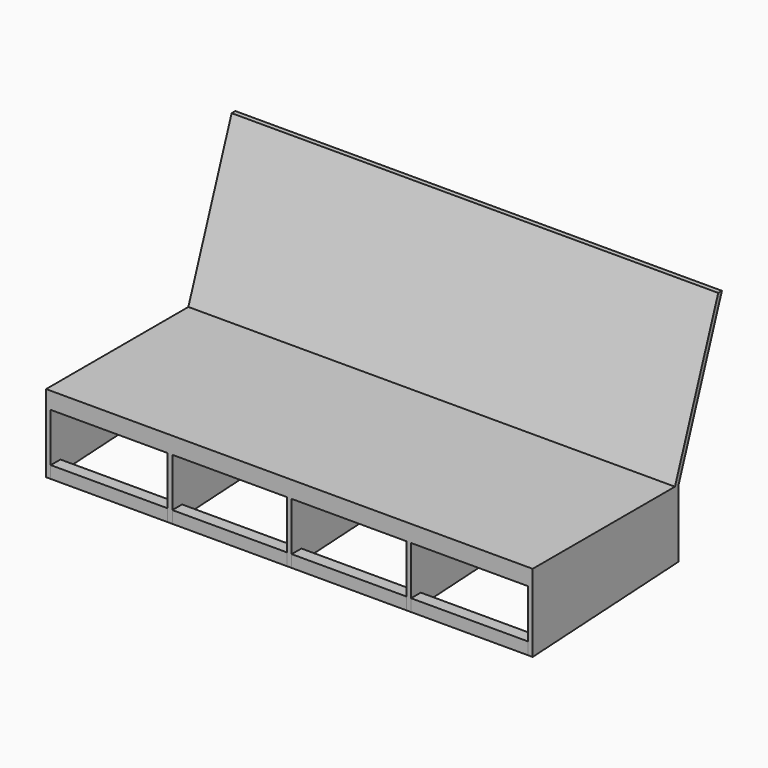
from build123d import *

# Parameters (mm, degrees)
F0_W       = 2000
F0_H       = 750
F1_DEPTH   = 19
F2_W       = 19
F2_H       = 750
F3_DEPTH   = 300
F4_SIZE2   = 39.99999
F4_SIZE    = 749.99999
F4_2_SIZE2 = 39.99999
F4_2_SIZE  = 749.99999
F4_3_SIZE2 = 39.99999
F4_3_SIZE  = 749.99999
F4_4_SIZE2 = 39.99999
F4_4_SIZE  = 749.99999
F4_5_SIZE2 = 39.99999
F4_5_SIZE  = 749.99999
F6_DEPTH   = 2000
F10_W      = 481
F10_H      = 50
F9_W       = 471.5
F9_H       = 50
F8_W       = 471.5
F8_H       = 50
F7_W       = 481
F7_H       = 50
F11_DEPTH  = 50
F12_W      = 50
F12_H      = 50
F13_DEPTH  = 2000


# Not quite as in the source:
# - a fillet or chamfer is up to 0.001 mm smaller than in the source, because OpenCascade refuses the exact size
# - ends of sketch curves that miss each other by under 0.0002 mm in the source are joined


with BuildPart() as f1:
    # F0 (on Top) → F1 (new body)
    with BuildSketch(Plane.XY):
        Rectangle(F0_W, F0_H)
    extrude(amount=F1_DEPTH)

    # F2 (on face) → F3 (join)
    with BuildSketch(Plane(origin=(0, 0, 0), x_dir=(1, 0, 0), z_dir=(0, 0, -1))):
        with Locations((-990.5, 0)):
            Rectangle(F2_W, F2_H)
        with Locations((-490.5, 0)):
            Rectangle(F2_W, F2_H)
        Rectangle(F2_W, F2_H)
        with Locations((490.5, 0)):
            Rectangle(F2_W, F2_H)
        with Locations((990.5, 0)):
            Rectangle(F2_W, F2_H)
    extrude(amount=F3_DEPTH)

    # F4 (size 750 and 40 in the source; OpenCascade refuses exactly that, so slightly less here)
    f4_edges = [f1.edges().sort_by_distance(p)[0] for p in [
        (990.5, 375, -300),
    ]]
    f4_side = f1.faces().sort_by_distance((990.5, 0, -300))[0]
    chamfer(f4_edges, length=F4_SIZE, length2=F4_SIZE2, reference=f4_side)

    # F4#2 (size 750 and 40 in the source; OpenCascade refuses exactly that, so slightly less here)
    f4_2_edges = [f1.edges().sort_by_distance(p)[0] for p in [
        (490.5, 375, -300),
    ]]
    f4_2_side = f1.faces().sort_by_distance((490.5, 0, -300))[0]
    chamfer(f4_2_edges, length=F4_2_SIZE, length2=F4_2_SIZE2, reference=f4_2_side)

    # F4#3 (size 750 and 40 in the source; OpenCascade refuses exactly that, so slightly less here)
    f4_3_edges = [f1.edges().sort_by_distance(p)[0] for p in [
        (0, 375, -300),
    ]]
    f4_3_side = f1.faces().sort_by_distance((0, 0, -300))[0]
    chamfer(f4_3_edges, length=F4_3_SIZE, length2=F4_3_SIZE2, reference=f4_3_side)

    # F4#4 (size 750 and 40 in the source; OpenCascade refuses exactly that, so slightly less here)
    f4_4_edges = [f1.edges().sort_by_distance(p)[0] for p in [
        (-490.5, 375, -300),
    ]]
    f4_4_side = f1.faces().sort_by_distance((-490.5, 0, -300))[0]
    chamfer(f4_4_edges, length=F4_4_SIZE, length2=F4_4_SIZE2, reference=f4_4_side)

    # F4#5 (size 750 and 40 in the source; OpenCascade refuses exactly that, so slightly less here)
    f4_5_edges = [f1.edges().sort_by_distance(p)[0] for p in [
        (-990.5, 375, -300),
    ]]
    f4_5_side = f1.faces().sort_by_distance((-990.5, 0, -300))[0]
    chamfer(f4_5_edges, length=F4_5_SIZE, length2=F4_5_SIZE2, reference=f4_5_side)

    # F5 (on face) → F6 (join)
    with BuildSketch(Plane(origin=(-1000, 0, 0), x_dir=(0, -1, 0), z_dir=(-1, 0, 0))):
        Polygon((-597.3130931617, 629.8002035108), (-375, 19), (-356, 19), (-578.3130931617, 629.8002035108), align=None)
    extrude(amount=-F6_DEPTH)

    # F10 (on face) + F9 (on face) + F8 (on face) + F7 (on face) → F11 (join)
    with BuildSketch(Plane(origin=(0, 0, 0), x_dir=(1, 0, 0), z_dir=(0, 0, -1))):
        with Locations((-740.5, 350)):
            Rectangle(F10_W, F10_H)
        with Locations((-740.5, -350)):
            Rectangle(F10_W, F10_H)
    with BuildSketch(Plane(origin=(0, 0, 0), x_dir=(1, 0, 0), z_dir=(0, 0, -1))):
        with Locations((-245.25, -350)):
            Rectangle(F9_W, F9_H)
        with Locations((-245.25, 350)):
            Rectangle(F9_W, F9_H)
    with BuildSketch(Plane(origin=(0, 0, 0), x_dir=(1, 0, 0), z_dir=(0, 0, -1))):
        with Locations((245.25, 350)):
            Rectangle(F8_W, F8_H)
        with Locations((245.25, -350)):
            Rectangle(F8_W, F8_H)
    with BuildSketch(Plane(origin=(0, 0, 0), x_dir=(1, 0, 0), z_dir=(0, 0, -1))):
        with Locations((740.5, 350)):
            Rectangle(F7_W, F7_H)
        with Locations((740.5, -350)):
            Rectangle(F7_W, F7_H)
    extrude(amount=F11_DEPTH)

    # F12 (on face) → F13 (join)
    with BuildSketch(Plane(origin=(-1000, 0, 0), x_dir=(0, -1, 0), z_dir=(-1, 0, 0))):
        with Locations((-350, -235)):
            Rectangle(F12_W, F12_H)
        Polygon((325, -250), (325, -297.3333344978), (374.99999, -300), (375, -250), align=None)
    extrude(amount=-F13_DEPTH)


solid = f1.part
